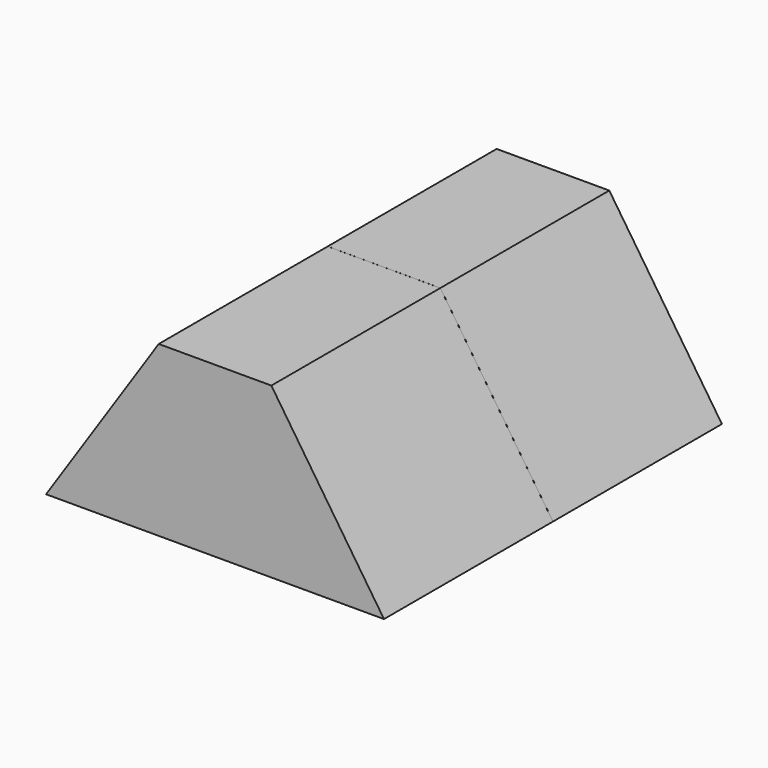
from build123d import *

# Parameters (mm, degrees)
F1_DEPTH  = 214.3125
F2_T      = -3.175
F4_DEPTH  = 3.175
F6_D      = 44.45
F6_DEPTH  = 3.175
F6_TIP    = 13.3541272579
F7_R      = 3.175
F8_DEPTH  = 25.4
F9_R      = 3.175
F10_DEPTH = 25.4
F5_R      = 1.5875
F11_DEPTH = 12.7
F12_R     = 4.7625
F12_R_2   = 3.175
F13_DEPTH = 1.5875
F14_W     = 171.45
F14_H     = 0.0254
F15_DEPTH = 85.725
F16_W     = 3.175
F16_H     = 3.175
F18_R     = 0.79375


with BuildPart() as f1:
    # F0 (on Front) → F1 (new body)
    with BuildSketch(Plane.XZ):
        Polygon((0, 42.8625), (0, -42.8625), (85.725, -42.8625), (28.575, 42.8625), align=None)
        Polygon((-28.575, 42.8625), (-85.725, -42.8625), (0, -42.8625), (0, 42.8625), align=None)
    extrude(amount=F1_DEPTH)

    # F2
    f2_openings = [f1.faces().sort_by_distance(p)[0] for p in [
        (0, 0, -7.14375),
    ]]
    offset(amount=F2_T, openings=f2_openings)

    # F3 (on Front) → F4 (join)
    with BuildSketch(Plane.XZ):
        Polygon((28.575, 42.8625), (-28.575, 42.8625), (-85.725, -42.8625), (85.725, -42.8625), align=None)
    extrude(amount=F4_DEPTH)

    # F6
    with Locations(Plane(origin=(0, 0, -42.8625), x_dir=(1, 0, 0), z_dir=(0, 0, -1))):
        with Locations((34.925, 50.8), (34.925, 163.5125)):
            Hole(F6_D / 2, depth=F6_DEPTH)
            with Locations((0, 0, -(F6_DEPTH + F6_TIP / 2))):  # 118° drill point
                Cone(0, F6_D / 2, F6_TIP, mode=Mode.SUBTRACT)

    # F7 (on face) → F8 (cut)
    with BuildSketch(Plane(origin=(0, 0, 0), x_dir=(-1, 0, 0), z_dir=(0, 1, 0))):
        with Locations((12.7, -12.7)):
            Circle(F7_R)
    extrude(amount=-F8_DEPTH, mode=Mode.SUBTRACT)

    # F9 (on face) → F10 (cut)
    with BuildSketch(Plane(origin=(0, 0, 0), x_dir=(-1, 0, 0), z_dir=(0, 1, 0))):
        with Locations((-12.7, -12.7)):
            Circle(F9_R)
    extrude(amount=-F10_DEPTH, mode=Mode.SUBTRACT)

    # F5 (on face) → F11 (cut)
    with BuildSketch(Plane(origin=(0, 0, -42.8625), x_dir=(1, 0, 0), z_dir=(0, 0, -1))):
        with Locations((57.15, 73.025)):
            Circle(F5_R)
        with Locations((57.15, 28.575)):
            Circle(F5_R)
        with Locations((12.7, 28.575)):
            Circle(F5_R)
        with Locations((12.7, 73.025)):
            Circle(F5_R)
        with Locations((12.7, 185.7375)):
            Circle(F5_R)
        with Locations((57.15, 185.7375)):
            Circle(F5_R)
        with Locations((57.15, 141.2875)):
            Circle(F5_R)
        with Locations((12.7, 141.2875)):
            Circle(F5_R)
    extrude(amount=-F11_DEPTH, mode=Mode.SUBTRACT)

    # F12 (on face) → F13 (cut)
    with BuildSketch(Plane.XZ.offset(3.175)):
        with Locations((12.7, -12.7)):
            Circle(F12_R)
        with Locations((12.7, -12.7)):
            Circle(F12_R_2, mode=Mode.SUBTRACT)
    extrude(amount=-F13_DEPTH, mode=Mode.SUBTRACT)

    # F14 (on face) → F15 (cut, through all)
    with BuildSketch(Plane(origin=(0, 0, -42.8625), x_dir=(1, 0, 0), z_dir=(0, 0, -1))):
        with Locations((0, 107.15625)):
            Rectangle(F14_W, F14_H)
    extrude(amount=-F15_DEPTH, mode=Mode.SUBTRACT)

    # F17: sweep along a path in F17_path
    with BuildLine(Plane(origin=(79.7924582335, -107.16895, -39.6875), x_dir=(0, 0, -1), z_dir=(0, 1, 0))) as f17_path:
        Line((0, 0), (0, 159.5849164669))
        Line((0, 159.5849164669), (-79.375, 106.6682498003))
        Line((-79.375, 106.6682498003), (-79.375, 52.9166666667))
        Line((-79.375, 52.9166666667), (0, 0))
    # F16 (on Right) → F17 (sweep)
    with BuildSketch(Plane.YZ):
        Polygon((-107.16895, -36.3601), (-111.134390904, -39.6875), (-107.16895, -39.6875), (-107.16895, -39.5351), align=None)
        with Locations((-105.58145, -37.9476)):
            Rectangle(F16_W, F16_H)
    sweep(path=f17_path.line, transition=Transition.RIGHT)

    # F18
    f18_edges = [f1.edges().sort_by_distance(p)[0] for p in [
        (-26.79423, -105.58145, 39.5351),
        (26.79423, -105.58145, 39.5351),
        (-79.507696, -105.58145, -39.5351),
        (79.507696, -105.58145, -39.5351),
    ]]
    fillet(f18_edges, radius=F18_R)


solid = f1.part
